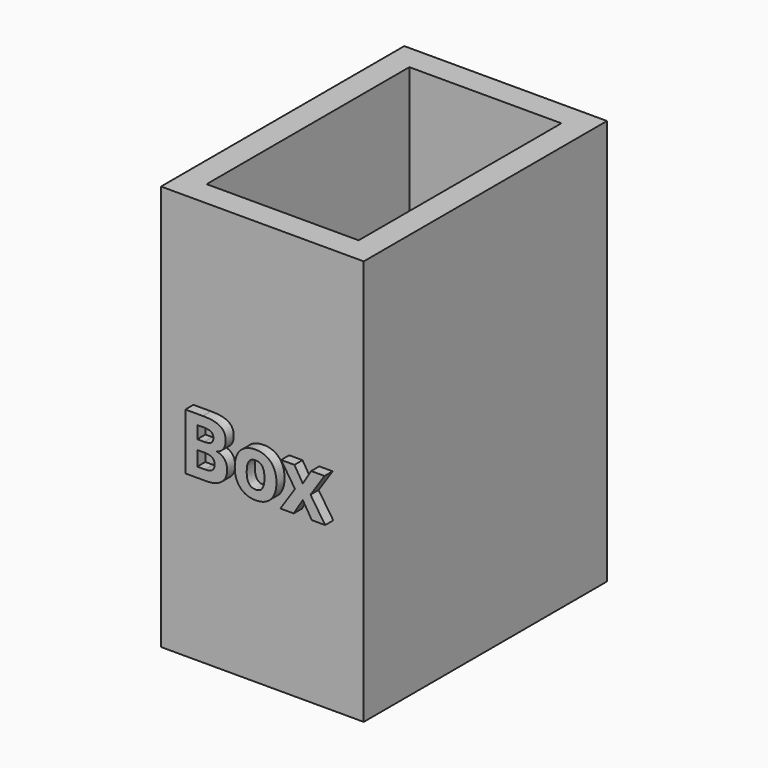
from build123d import *

# Parameters (mm, degrees)
F0_W         = 50.8
F0_H         = 101.6
F1_DEPTH     = 76.2
F2_T         = -6.35
F3_TEXT_SIZE = 19.7489268648
F4_DEPTH     = 2.54


# Not quite as in the source:
# - Text() gives the source's letters only with a copy of the font that has no kerning and outlines rounded to 1/6400 em; it was checked with that copy


with BuildPart() as f1:
    # F0 (on Front) → F1 (new body)
    with BuildSketch(Plane.XZ):
        with Locations((-24.2544179782, 26.6049756312)):
            Rectangle(F0_W, F0_H)
    extrude(amount=F1_DEPTH)

    # F2
    f2_openings = [f1.faces().sort_by_distance(p)[0] for p in [
        (-24.254418, -38.1, 77.404976),
    ]]
    offset(amount=F2_T, openings=f2_openings)

    # F3 (on face) → F4 (join)
    with BuildSketch(Plane.XZ.offset(76.2)):
        with Locations((-43.3044179782, 17.7830829865)):
            Text('Box', F3_TEXT_SIZE, font='Open Sans', font_style=FontStyle.BOLD, text_align=(TextAlign.LEFT, TextAlign.BOTTOM))
    extrude(amount=F4_DEPTH)


solid = f1.part
